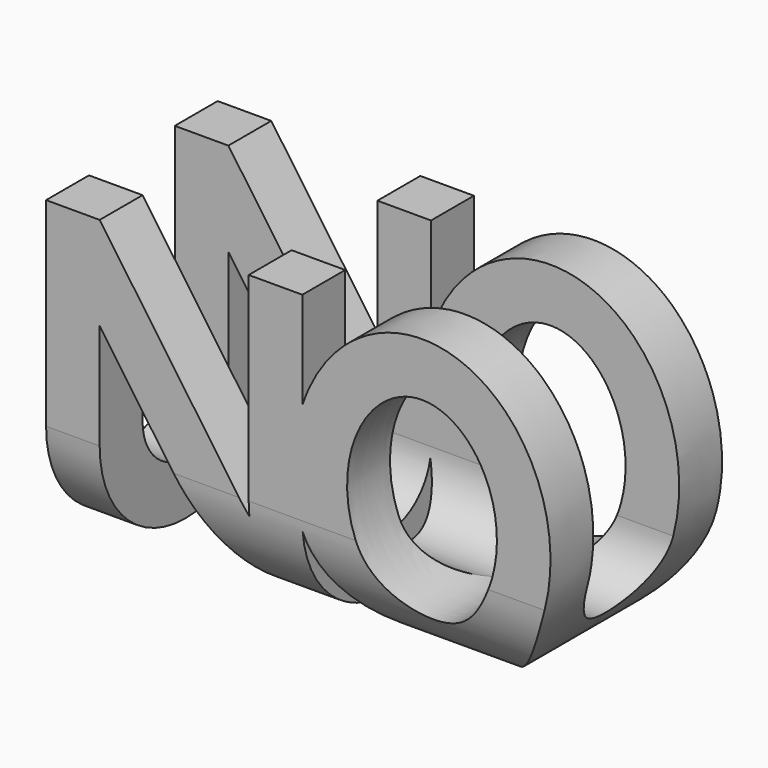
from build123d import *

# Parameters (mm, degrees)
F1_DEPTH = 50.8
F3_START = -41.830430107
F3_DEPTH = 83.6608602141


# Not quite as in the source:
# - the dataset's text gives a spline's control points without its knots; the knots are read off the source's solid


with BuildPart() as f1:
    # F0 (on Front) → F1 (new body, symmetric)
    with BuildSketch(Plane.XZ):
        with BuildLine():
            add(Edge.make_bspline(
                [(0.6684268399, -9.2552149613), (7.1062361508, -28.8634498325), (24.4678330789, -24.9596258419), (41.829430007, -21.0558018514), (41.829430007, 0)],
                knots=[1.9437617056, 1.9437617056, 1.9437617056, 3.328075343, 3.328075343, 4.7123889804, 4.7123889804, 4.7123889804], degree=2, weights=[1, 0.7698713269, 1, 0.7698713269, 1]))
            add(Edge.make_bspline(
                [(41.829430007, 0), (41.829430007, 21.0558018514), (24.4678330789, 24.9596258419), (7.1062361508, 28.8634498325), (0.6684268399, 9.2552149613)],
                knots=[4.7123889804, 4.7123889804, 4.7123889804, 6.0967026178, 6.0967026178, 7.4810162551, 7.4810162551, 7.4810162551], degree=2, weights=[1, 0.7698713269, 1, 0.7698713269, 1]))
            Line((0.6684268399, 9.2552149613), (0.6684268399, -9.2552149613))
        make_face()
        with BuildLine():
            add(Edge.make_bspline(
                [(20.5162993751, 16.51), (20.1618438648, 16.51), (19.4529328442, 16.4680414875), (18.3990854052, 16.2806728015), (17.3456301166, 15.965854662), (15.9439052846, 15.3689450051), (14.5532102117, 14.4922507846), (13.213807035, 13.313724527), (12.2450650285, 12.2704531887), (11.3405845091, 11.0812450704), (10.5259351491, 9.7704064229), (9.8091298744, 8.3438600703), (9.2027224088, 6.8159749061), (8.7169570858, 5.2014498103), (8.3610826846, 3.5167170688), (8.1791763521, 2.0679821858), (8.1055695228, 0.891126151), (8.0869683535, 0), (8.1055695228, -0.891126151), (8.1791763521, -2.0679821858), (8.3610826846, -3.5167170688), (8.7169570858, -5.2014498103), (9.2027224088, -6.8159749061), (9.8091298744, -8.3438600703), (10.5259351491, -9.7704064229), (11.3405845091, -11.0812450704), (12.2450650285, -12.2704531887), (13.213807035, -13.313724527), (14.5532102117, -14.4922507846), (15.9439052846, -15.3689450051), (17.3456301166, -15.965854662), (18.3990854052, -16.2806728015), (19.4529328442, -16.4680414875), (20.5162993751, -16.5309792562), (21.5796659061, -16.4680414875), (22.6335133451, -16.2806728015), (23.6869686337, -15.965854662), (25.0886934657, -15.3689450051), (26.4793885386, -14.4922507846), (27.8187917153, -13.313724527), (28.7875337218, -12.2704531887), (29.6920142412, -11.0812450704), (30.5066636012, -9.7704064229), (31.2234688759, -8.3438600703), (31.8298763415, -6.8159749061), (32.3156416645, -5.2014498103), (32.6715160657, -3.5167170688), (32.8534223982, -2.0679821858), (32.9270292275, -0.891126151), (32.9456303968, 0), (32.9270292275, 0.891126151), (32.8534223982, 2.0679821858), (32.6715160657, 3.5167170688), (32.3156416645, 5.2014498103), (31.8298763415, 6.8159749061), (31.2234688759, 8.3438600703), (30.5066636012, 9.7704064229), (29.6920142412, 11.0812450704), (28.7875337218, 12.2704531887), (27.8187917153, 13.313724527), (26.4793885386, 14.4922507846), (25.0886934657, 15.3689450051), (23.6869686337, 15.965854662), (22.6335133451, 16.2806728015), (21.5796659061, 16.4680414875), (20.8707548855, 16.51), (20.5162993751, 16.51)],
                knots=[0, 0, 0, 0, 0.015625, 0.03125, 0.046875, 0.0625, 0.09375, 0.109375, 0.125, 0.140625, 0.15625, 0.171875, 0.1875, 0.203125, 0.21875, 0.234375, 0.2421875, 0.25, 0.2578125, 0.265625, 0.28125, 0.296875, 0.3125, 0.328125, 0.34375, 0.359375, 0.375, 0.390625, 0.40625, 0.4375, 0.453125, 0.46875, 0.484375, 0.5, 0.515625, 0.53125, 0.546875, 0.5625, 0.59375, 0.609375, 0.625, 0.640625, 0.65625, 0.671875, 0.6875, 0.703125, 0.71875, 0.734375, 0.7421875, 0.75, 0.7578125, 0.765625, 0.78125, 0.796875, 0.8125, 0.828125, 0.84375, 0.859375, 0.875, 0.890625, 0.90625, 0.9375, 0.953125, 0.96875, 0.984375, 1, 1, 1, 1], degree=3))
        make_face(mode=Mode.SUBTRACT)
        with BuildLine():
            Line((0.6684268399, -9.2552149613), (0.6684268399, 9.2552149613))
            add(Edge.make_bspline(
                [(0.6684268399, 9.2552149613), (-2.3702612135, 0), (0.6684268399, -9.2552149613)],
                knots=[1.1978309479, 1.1978309479, 1.1978309479, 1.9437617056, 1.9437617056, 1.9437617056], degree=2, weights=[1, 0.9312509212, 1]))
        make_face()
        with BuildLine():
            add(Edge.make_bspline(
                [(0.6684268399, 9.2552149613), (-2.3702612135, 0), (0.6684268399, -9.2552149613)],
                knots=[1.1978309479, 1.1978309479, 1.1978309479, 1.9437617056, 1.9437617056, 1.9437617056], degree=2, weights=[1, 0.9312509212, 1]))
            Line((0.6684268399, 9.2552149613), (0.6684268399, 25.4))
            Line((0.6684268399, 25.4), (-8.2215731601, 25.4))
            Line((-8.2215731601, 25.4), (-8.2215731601, -9.9007579869))
            Line((-8.2215731601, -9.9007579869), (-32.939430007, 25.4))
            Line((-32.939430007, 25.4), (-41.829430007, 25.4))
            Line((-41.829430007, 25.4), (-41.829430007, -25.4))
            Line((-41.829430007, -25.4), (-32.939430007, -25.4))
            Line((-32.939430007, -25.4), (-32.939430007, 9.9007579869))
            Line((-32.939430007, 9.9007579869), (-8.2215731601, -25.4))
            Line((-8.2215731601, -25.4), (0.6684268399, -25.4))
            Line((0.6684268399, -25.4), (0.6684268399, -9.2552149613))
        make_face()
    extrude(amount=F1_DEPTH, both=True)

    # F2 (on Right) → F3 (intersect)
    with BuildSketch(Plane.YZ.offset(F3_START)):
        with BuildLine():
            Line((-8.8952714705, 25.4), (-17.7852714705, 25.4))
            Line((-17.7852714705, 25.4), (-17.7852714705, -7.6147285295))
            ThreePointArc((-17.7852714705, -7.6147285295), (0, -25.4), (17.7852714705, -7.6147285295))
            Line((17.7852714705, -7.6147285295), (17.7852714705, 25.4))
            Line((17.7852714705, 25.4), (8.8952714705, 25.4))
            Line((8.8952714705, 25.4), (8.8952714705, -7.6147285295))
            ThreePointArc((8.8952714705, -7.6147285295), (0, -16.51), (-8.8952714705, -7.6147285295))
            Line((-8.8952714705, -7.6147285295), (-8.8952714705, 25.4))
        make_face()
    extrude(amount=F3_DEPTH, mode=Mode.INTERSECT)


solid = f1.part
